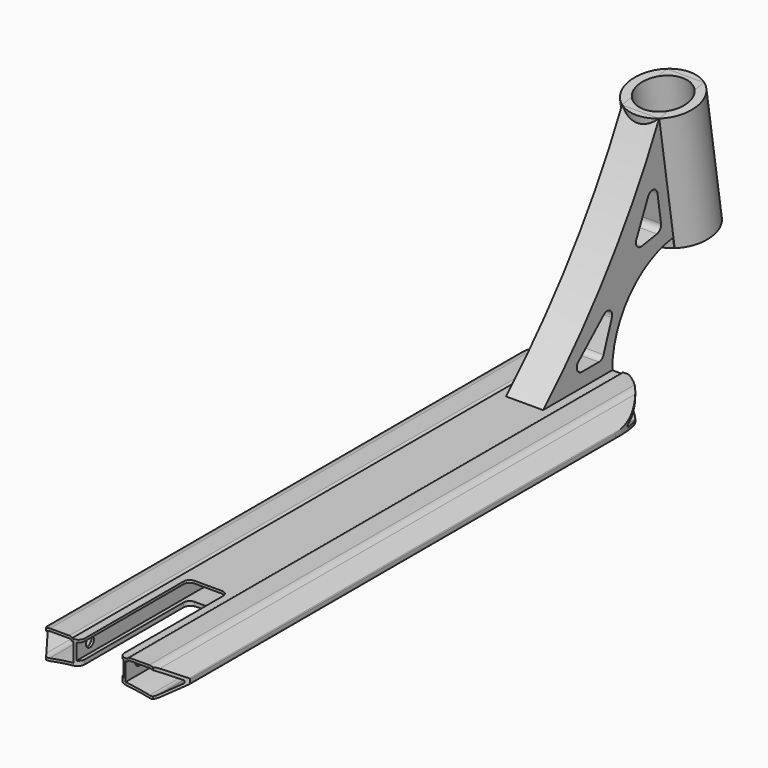
from build123d import *

# Parameters (mm, degrees)
F1_DEPTH       = 250
F2_W           = 38
F2_H           = 13
F3_DEPTH       = 528
F4_R           = 9
F5_R           = 1
F6_T1_DEPTH    = 509.3674969976
F8_DEPTH       = 500.001
F10_DEPTH      = 526
F10_DEPTH_BACK = 24.001
F12_DEPTH      = 527
F12_DEPTH_BACK = 24.0010001
F13_T1_DEPTH   = 2
F13_T6_DEPTH   = 32
F13_S7_R       = 200
F13_T8_DEPTH   = 18
F13_T13_DEPTH  = 33.5797498408
F13_S14_R      = 200
F13_T15_DEPTH  = 19
F13_T19_DEPTH  = 63.5797498408
F13_T25_DEPTH  = 32
F13_S26_R      = 200
F13_T27_DEPTH  = 18
F13_T32_DEPTH  = 33.5797498408
F13_S33_R      = 200
F13_T34_DEPTH  = 19
F13_T38_DEPTH  = 63.5797498408
F13_T41_DEPTH  = 62
F13_T43_DEPTH  = 63.5797498408
F15_DEPTH      = 15
F16_R          = 27.5
F17_DEPTH      = 100
F20_D          = 40
F21_D          = 8
F21_DEPTH      = 50
F21_TIP        = 2.4034424761
F23_DEPTH      = 72.5010001
F24_R          = 5


# Not quite as in the source:
# - a fillet or chamfer that OpenCascade refuses, or shapes differently, is made with other operations: its cross-section is extruded or revolved along the edge and cut away or added
# - an extrude ends at something that could not be found from the text; its depth is read off the source's solid


with BuildPart() as f1:
    # F0 (on Front) → F1 (new body, symmetric)
    with BuildSketch(Plane.XZ):
        with BuildLine():
            Line((57.5, 8.1520738932), (57.5, 12.1520738932))
            Line((57.5, 12.1520738932), (43.3801914974, 24))
            Line((43.3801914974, 24), (22.5, 24))
            Line((22.5, 24), (22.5, 22.7))
            Line((22.5, 22.7), (0, 22.7))
            Line((0, 22.7), (-22.5, 22.7))
            Line((-22.5, 22.7), (-22.5, 24))
            Line((-22.5, 24), (-43.3801914974, 24))
            Line((-43.3801914974, 24), (-57.5, 12.1520738932))
            Line((-57.5, 12.1520738932), (-57.5, 8.1520738932))
            Line((-57.5, 8.1520738932), (-43.3801938299, 0))
            ThreePointArc((-43.3801938299, 0), (0, 4.7612774492), (43.3801938299, 0))
            Line((43.3801938299, 0), (57.5, 8.1520738932))
        make_face()
    extrude(amount=F1_DEPTH, both=True)

    # F2 (on face) → F3 (cut, symmetric)
    with BuildSketch(Plane.XZ.offset(250)):
        with Locations((0, 14.2)):
            Rectangle(F2_W, F2_H)
    extrude(amount=F3_DEPTH, both=True, mode=Mode.SUBTRACT)

    # F4
    f4_edges = [f1.edges().sort_by_distance(p)[0] for p in [
        (-43.380191, 0, 24),
        (-43.380194, 0, 0),
        (43.380191, 0, 24),
        (43.380194, 0, 0),
    ]]
    fillet(f4_edges, radius=F4_R)

    # F5
    f5_edges = [f1.edges().sort_by_distance(p)[0] for p in [
        (-57.5, 0, 12.152074),
        (-57.5, 0, 8.152074),
        (57.5, 0, 12.152074),
        (57.5, 0, 8.152074),
    ]]
    fillet(f5_edges, radius=F5_R)

    # F6: fillet of radius 2 on 2 edges, made by hand

    # F6_s2 → F6_t1 (cut)
    with BuildSketch(Plane.XZ.offset(-254.6837484988)):
        with BuildLine():
            ThreePointArc((-24.3734993995, 24), (-23.2333239744, 23.6431676725), (-22.5, 22.7))
            Line((-22.5, 22.7), (-22.5, 24))
            Line((-22.5, 24), (-24.3734993995, 24))
        make_face()
        with BuildLine():
            ThreePointArc((22.5, 22.7), (23.2333239744, 23.6431676725), (24.3734993995, 24))
            Line((24.3734993995, 24), (22.5, 24))
            Line((22.5, 24), (22.5, 22.7))
        make_face()
    extrude(amount=F6_T1_DEPTH, mode=Mode.SUBTRACT)

    # F7 (on face) → F8 (cut, through all)
    with BuildSketch(Plane.XZ.offset(250)):
        with BuildLine():
            ThreePointArc((-40.4725072541, 2.6652343489), (-30.7728699967, 4.4035336781), (-21, 5.6667278481))
            Line((-21, 5.6667278481), (-21, 7.7))
            Line((-21, 7.7), (-21, 20.7))
            Line((-21, 20.7), (-22.5, 20.7))
            ThreePointArc((-22.5, 20.7), (-23.2333239744, 21.6431676725), (-24.3734993995, 22))
            Line((-24.3734993995, 22), (-40.1044593891, 22))
            ThreePointArc((-40.1044593891, 22), (-42.4986003923, 21.5778483455), (-44.6039726569, 20.3623111018))
            Line((-44.6039726569, 20.3623111018), (-55.1427876097, 11.5191953619))
            ThreePointArc((-55.1427876097, 11.5191953619), (-55.406307787, 11.1757691805), (-55.5, 10.7531509187))
            Line((-55.5, 10.7531509187), (-55.5, 9.8841247008))
            ThreePointArc((-55.5, 9.8841247008), (-55.3660254038, 9.3841247008), (-55, 9.018099297))
            Line((-55, 9.018099297), (-45.3750198817, 3.4611144348))
            ThreePointArc((-45.3750198817, 3.4611144348), (-42.9967237629, 2.6137495555), (-40.4725072541, 2.6652343489))
        make_face()
        with BuildLine():
            ThreePointArc((21, 5.6667278481), (30.7728699967, 4.4035336781), (40.4725072541, 2.6652343489))
            ThreePointArc((40.4725072541, 2.6652343489), (42.9967237629, 2.6137495555), (45.3750198817, 3.4611144348))
            Line((45.3750198817, 3.4611144348), (55, 9.018099297))
            ThreePointArc((55, 9.018099297), (55.3660254038, 9.3841247008), (55.5, 9.8841247008))
            Line((55.5, 9.8841247008), (55.5, 10.7531509187))
            ThreePointArc((55.5, 10.7531509187), (55.406307787, 11.1757691805), (55.1427876097, 11.5191953619))
            Line((55.1427876097, 11.5191953619), (44.6039726569, 20.3623111018))
            ThreePointArc((44.6039726569, 20.3623111018), (42.4986003923, 21.5778483455), (40.1044593891, 22))
            Line((40.1044593891, 22), (24.3734993995, 22))
            ThreePointArc((24.3734993995, 22), (23.2333239744, 21.6431676725), (22.5, 20.7))
            Line((22.5, 20.7), (21, 20.7))
            Line((21, 20.7), (21, 7.7))
            Line((21, 7.7), (21, 5.6667278481))
        make_face()
    extrude(amount=-F8_DEPTH, mode=Mode.SUBTRACT)

    # F9 (on Top) → F10 (cut, two sides)
    with BuildSketch(Plane.XY) as f10_sk:
        with BuildLine():
            ThreePointArc((-57.5, 200), (0, 257.5), (57.5, 200))
            Line((57.5, 200), (57.5, 280))
            Line((57.5, 280), (-57.5, 280))
            Line((-57.5, 280), (-57.5, 200))
        make_face()
    extrude(amount=-F10_DEPTH, mode=Mode.SUBTRACT)
    extrude(f10_sk.sketch, amount=F10_DEPTH_BACK, mode=Mode.SUBTRACT)

    # F11 (on Top) → F12 (cut, two sides)
    with BuildSketch(Plane.XY) as f12_sk:
        Polygon((-68, -216), (-68, -346), (68, -346), (68, -216), (43.2975540478, -250), (16, -250), (16, -140), (-16, -140), (-16, -250), (-43.2975540478, -250), align=None)
    extrude(amount=-F12_DEPTH, mode=Mode.SUBTRACT)
    extrude(f12_sk.sketch, amount=F12_DEPTH_BACK, mode=Mode.SUBTRACT)

    # F13: fillet of radius 5 on 6 edges, made by hand

    # F13_s2 → F13_t1 (join)
    with BuildSketch(Plane.XY.offset(20.7)):
        with BuildLine():
            ThreePointArc((-11, -140), (-14.5355339059, -141.4644660941), (-16, -145))
            Line((-16, -145), (-16.1, -145))
            Line((-16.1, -145), (-16.1, -139.9))
            Line((-16.1, -139.9), (-11, -139.9))
            Line((-11, -139.9), (-11, -140))
        make_face()
        with BuildLine():
            ThreePointArc((16, -145), (14.5355339059, -141.4644660941), (11, -140))
            Line((11, -140), (11, -139.9))
            Line((11, -139.9), (16.1, -139.9))
            Line((16.1, -139.9), (16.1, -145))
            Line((16.1, -145), (16, -145))
        make_face()
    extrude(amount=F13_T1_DEPTH)


with BuildPart() as f13_tool4:
    # F13_s5 → F13_t6 (new body)
    with BuildSketch(Plane.XY.offset(-9.3)):
        with BuildLine():
            ThreePointArc((-11, -140), (-14.5355339059, -141.4644660941), (-16, -145))
            Line((-16, -145), (-16.1, -145))
            Line((-16.1, -145), (-16.1, -139.9))
            Line((-16.1, -139.9), (-11, -139.9))
            Line((-11, -139.9), (-11, -140))
        make_face()
    extrude(amount=F13_T6_DEPTH)

    # F13_s7 → F13_t8 (cut, symmetric)
    with BuildSketch(Plane.XZ.offset(142.4)):
        with Locations((0, -195.2387225508)):
            Circle(F13_S7_R)
    extrude(amount=F13_T8_DEPTH, both=True, mode=Mode.SUBTRACT)

    split(bisect_by=Plane.XY.offset(7.7), keep=Keep.BOTTOM)


with BuildPart() as f1_1:
    add(f1.part)

    # F13_t3: union F13_tool4
    add(f13_tool4.part)


with BuildPart() as f13_tool11:
    # F13_s12 → F13_t13 (new body)
    with BuildSketch(Plane.XY.offset(-25.8797498408)):
        with BuildLine():
            ThreePointArc((-16, -145), (-14.5355339059, -141.4644660941), (-11, -140))
            Line((-11, -140), (-11, -139.9))
            Line((-11, -139.9), (-16.1, -139.9))
            Line((-16.1, -139.9), (-16.1, -145))
            Line((-16.1, -145), (-16, -145))
        make_face()
    extrude(amount=F13_T13_DEPTH)

    # F13_s14 → F13_t15 (cut, symmetric)
    with BuildSketch(Plane.XZ.offset(142.4)):
        with Locations((0, -195.2387225508)):
            Circle(F13_S14_R)
    extrude(amount=F13_T15_DEPTH, both=True, mode=Mode.SUBTRACT)


with BuildPart() as f1_2:
    add(f1_1.part)

    # F13_t10: union F13_tool11
    add(f13_tool11.part)


with BuildPart() as f13_tool17:
    # F13_s18 → F13_t19 (new body)
    with BuildSketch(Plane.XY.offset(-25.8797498408)):
        with BuildLine():
            ThreePointArc((-16, -145), (-14.5355339059, -141.4644660941), (-11, -140))
            Line((-11, -140), (-11, -139.9))
            Line((-11, -139.9), (-16.1, -139.9))
            Line((-16.1, -139.9), (-16.1, -145))
            Line((-16.1, -145), (-16, -145))
        make_face()
    extrude(amount=F13_T19_DEPTH)

    split(bisect_by=Plane.XY.offset(22.7), keep=Keep.BOTTOM)

    split(bisect_by=Plane.XY.offset(20.7), keep=Keep.TOP)


with BuildPart() as f1_3:
    add(f1_2.part)

    # F13_t16: union F13_tool17
    add(f13_tool17.part)


with BuildPart() as f13_tool23:
    # F13_s24 → F13_t25 (new body)
    with BuildSketch(Plane.XY.offset(-9.3)):
        with BuildLine():
            ThreePointArc((16, -145), (14.5355339059, -141.4644660941), (11, -140))
            Line((11, -140), (11, -139.9))
            Line((11, -139.9), (16.1, -139.9))
            Line((16.1, -139.9), (16.1, -145))
            Line((16.1, -145), (16, -145))
        make_face()
    extrude(amount=F13_T25_DEPTH)

    # F13_s26 → F13_t27 (cut, symmetric)
    with BuildSketch(Plane.XZ.offset(142.4)):
        with Locations((0, -195.2387225508)):
            Circle(F13_S26_R)
    extrude(amount=F13_T27_DEPTH, both=True, mode=Mode.SUBTRACT)

    split(bisect_by=Plane.XY.offset(7.7), keep=Keep.BOTTOM)


with BuildPart() as f1_4:
    add(f1_3.part)

    # F13_t22: union F13_tool23
    add(f13_tool23.part)


with BuildPart() as f13_tool30:
    # F13_s31 → F13_t32 (new body)
    with BuildSketch(Plane.XY.offset(-25.8797498408)):
        with BuildLine():
            ThreePointArc((11, -140), (14.5355339059, -141.4644660941), (16, -145))
            Line((16, -145), (16.1, -145))
            Line((16.1, -145), (16.1, -139.9))
            Line((16.1, -139.9), (11, -139.9))
            Line((11, -139.9), (11, -140))
        make_face()
    extrude(amount=F13_T32_DEPTH)

    # F13_s33 → F13_t34 (cut, symmetric)
    with BuildSketch(Plane.XZ.offset(142.4)):
        with Locations((0, -195.2387225508)):
            Circle(F13_S33_R)
    extrude(amount=F13_T34_DEPTH, both=True, mode=Mode.SUBTRACT)


with BuildPart() as f1_5:
    add(f1_4.part)

    # F13_t29: union F13_tool30
    add(f13_tool30.part)


with BuildPart() as f13_tool36:
    # F13_s37 → F13_t38 (new body)
    with BuildSketch(Plane.XY.offset(-25.8797498408)):
        with BuildLine():
            ThreePointArc((11, -140), (14.5355339059, -141.4644660941), (16, -145))
            Line((16, -145), (16.1, -145))
            Line((16.1, -145), (16.1, -139.9))
            Line((16.1, -139.9), (11, -139.9))
            Line((11, -139.9), (11, -140))
        make_face()
    extrude(amount=F13_T38_DEPTH)

    split(bisect_by=Plane.XY.offset(22.7), keep=Keep.BOTTOM)

    split(bisect_by=Plane.XY.offset(20.7), keep=Keep.TOP)


with BuildPart() as f1_6:
    add(f1_5.part)

    # F13_t35: union F13_tool36
    add(f13_tool36.part)

    # F13_s42 → F13_t41 (cut)
    with BuildSketch(Plane.XY.offset(-9.3)):
        with BuildLine():
            ThreePointArc((-21, -250), (-17.4644660941, -248.5355339059), (-16, -245))
            Line((-16, -245), (-15.9, -245))
            Line((-15.9, -245), (-15.9, -250.1))
            Line((-15.9, -250.1), (-21, -250.1))
            Line((-21, -250.1), (-21, -250))
        make_face()
    extrude(amount=F13_T41_DEPTH, mode=Mode.SUBTRACT)

    # F13_s44 → F13_t43 (cut)
    with BuildSketch(Plane.XY.offset(-25.8797498408)):
        with BuildLine():
            ThreePointArc((21, -250), (17.4644660941, -248.5355339059), (16, -245))
            Line((16, -245), (15.9, -245))
            Line((15.9, -245), (15.9, -250.1))
            Line((15.9, -250.1), (21, -250.1))
            Line((21, -250.1), (21, -250))
        make_face()
    extrude(amount=F13_T43_DEPTH, mode=Mode.SUBTRACT)

    # F14 (on Right) → F15 (join, symmetric)
    with BuildSketch(Plane.YZ):
        with BuildLine():
            ThreePointArc((297.3819995028, 182.7), (245.9666940414, 97.362277853), (180, 22.7))
            Line((180, 22.7), (250, 22.7))
            ThreePointArc((250, 22.7), (267.6550746197, 69.1758946867), (311.7145367693, 92.2079211245))
            Line((311.7145367693, 92.2079211245), (313.0254460068, 83.9311659405))
            Line((313.0254460068, 83.9311659405), (358.4591096742, 91.1271513323))
            Line((358.4591096742, 91.1271513323), (342.8156631702, 189.8959853919))
            Line((342.8156631702, 189.8959853919), (297.3819995028, 182.7))
        make_face()
    extrude(amount=F15_DEPTH, both=True)

    # F16 (on face) → F17 (join, through all)
    with BuildSketch(Plane(origin=(0, -20.9512469128, 132.2809669298), x_dir=(1, 0, 0), z_dir=(0, -0.156434465, 0.9876883406))):
        with Locations((0, 345.5046751792)):
            Circle(F16_R)
    extrude(amount=-F17_DEPTH)

    # F20 (through all)
    with Locations(Plane(origin=(0, -20.9512469128, 132.2809669298), x_dir=(1, 0, 0), z_dir=(0, -0.156434465, 0.9876883406))):
        with Locations((0, 345.5046751792)):
            Hole(F20_D / 2)

    # F21 (one way)
    with BuildSketch(Plane.YZ.offset(21)):
        with Locations((-236, 15.6667278481)):
            Circle(F21_D / 2)
    extrude(amount=-F21_DEPTH, mode=Mode.SUBTRACT)
    with Locations(Plane.YZ.offset(21)):
        with Locations((-236, 15.6667278481)):
            with Locations((0, 0, -(F21_DEPTH + F21_TIP / 2))):  # 118° drill point
                Cone(0, F21_D / 2, F21_TIP, mode=Mode.SUBTRACT)

    # F22 (on face) → F23 (cut, through all)
    with BuildSketch(Plane.YZ.offset(15)):
        Polygon((256.378660542, 79), (206, 34), (240, 34), align=None)
        Polygon((293.1329238381, 146.5907331264), (270.5418245471, 97.4517238484), (300.1724747649, 102.1447577996), align=None)
    extrude(amount=-F23_DEPTH, mode=Mode.SUBTRACT)

    # F24
    f24_edges = [f1_6.edges().sort_by_distance(p)[0] for p in [
        (0, 300.172475, 102.144758),
        (0, 270.541825, 97.451724),
        (0, 293.132924, 146.590733),
        (0, 256.378661, 79),
        (0, 240, 34),
        (0, 206, 34),
    ]]
    fillet(f24_edges, radius=F24_R)


solid = f1_6.part
